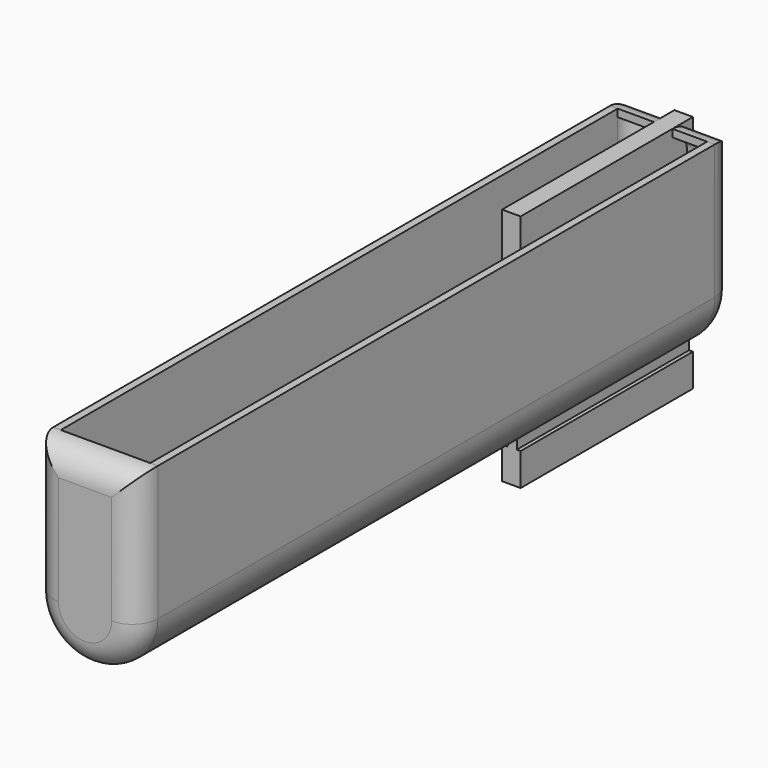
from build123d import *

# Parameters (mm, degrees)
F0_W      = 35
F0_H      = 250
F1_DEPTH  = 45
F3_DEPTH  = 250
F4_DEPTH  = 250
F5_R      = 8.5849434278
F6_T      = -2.54
F7_W      = 6.1992760748
F7_H      = 72.0517709851
F8_DEPTH  = 80
F10_DEPTH = 101.346


# Not quite as in the source:
# - a shell that OpenCascade refuses in one call is made with other operations: the cavity is built on its own and cut out
# - a feature names something its author has since deleted; it is built from what else it names


with BuildPart() as f1:
    # F0 (on Top) → F1 (new body)
    with BuildSketch(Plane.XY):
        with Locations((17.5, -125)):
            Rectangle(F0_W, F0_H)
    extrude(amount=-F1_DEPTH)

    # F2 (on face) → F3 (join)
    with BuildSketch(Plane(origin=(0, 0, 0), x_dir=(-1, 0, 0), z_dir=(0, 1, 0))):
        with BuildLine():
            Line((-17.5, -45), (0, -45))
            ThreePointArc((0, -45), (-5.1256313292, -32.6256313292), (-17.5, -27.5))
            ThreePointArc((-17.5, -27.5), (-29.8743686708, -32.6256313292), (-35, -45))
            Line((-35, -45), (-17.5, -45))
        make_face()
        with BuildLine():
            ThreePointArc((-35, -45), (-17.5, -62.5), (0, -45))
            Line((0, -45), (-17.5, -45))
            Line((-17.5, -45), (-35, -45))
        make_face()
        with BuildLine():
            ThreePointArc((-17.5, -27.5), (-5.1256313292, -32.6256313292), (0, -45))
            Line((0, -45), (0, -27.5))
            Line((0, -27.5), (-17.5, -27.5))
        make_face()
    extrude(amount=-F3_DEPTH)

    # F2 (on face) → F4 (join)
    with BuildSketch(Plane(origin=(0, 0, 0), x_dir=(-1, 0, 0), z_dir=(0, 1, 0))):
        with BuildLine():
            Line((-17.5, -45), (0, -45))
            ThreePointArc((0, -45), (-5.1256313292, -32.6256313292), (-17.5, -27.5))
            ThreePointArc((-17.5, -27.5), (-29.8743686708, -32.6256313292), (-35, -45))
            Line((-35, -45), (-17.5, -45))
        make_face()
        with BuildLine():
            ThreePointArc((-35, -45), (-17.5, -62.5), (0, -45))
            Line((0, -45), (-17.5, -45))
            Line((-17.5, -45), (-35, -45))
        make_face()
        with BuildLine():
            ThreePointArc((-17.5, -27.5), (-5.1256313292, -32.6256313292), (0, -45))
            Line((0, -45), (0, -27.5))
            Line((0, -27.5), (-17.5, -27.5))
        make_face()
    extrude(amount=-F4_DEPTH)

    # F5
    f5_edges = [f1.edges().sort_by_distance(p)[0] for p in [
        (17.5, 0, 0),
        (35, 0, -22.5),
        (17.5, 0, -62.5),
        (0, 0, -22.5),
        (17.5, -250, 0),
        (0, -250, -22.5),
        (17.5, -250, -62.5),
        (35, -250, -22.5),
    ]]
    fillet(f5_edges, radius=F5_R)

    # F6: a shell. OpenCascade refuses it in one call, so the cavity is built on its own and cut out:
    # the body offset inwards by the wall thickness, plus a prism from it out through each open face.
    f6_core = offset(f1.part, amount=F6_T, mode=Mode.PRIVATE)
    f6_exits = [f6_core.faces().sort_by_distance(p)[0] for p in [
        (17.5, -125, -2.54),
    ]]
    add(f6_core, mode=Mode.SUBTRACT)
    extrude(f6_exits, amount=-F6_T, mode=Mode.SUBTRACT)

    # F7 (on Top) → F8 (join)
    with BuildSketch(Plane.XY):
        with Locations((17.7442375571, -36.0258854926)):
            Rectangle(F7_W, F7_H)
    extrude(amount=-F8_DEPTH)

    # F9 (on face) → F10 (cut)
    with BuildSketch(Plane.XZ.offset(72.0517709851)):
        Polygon((16.4569599832, -69.1932439804), (16.4569599832, -62.46888856), (14.6445995197, -62.5368878245), (14.6445995197, -69.1932439804), align=None)
        Polygon((20.8438755944, -62.1775579175), (19.5716265936, -62.376949193), (19.5716265936, -69.1005588385), (20.8438755944, -69.1005588385), align=None)
    extrude(amount=-F10_DEPTH, mode=Mode.SUBTRACT)


solid = f1.part
